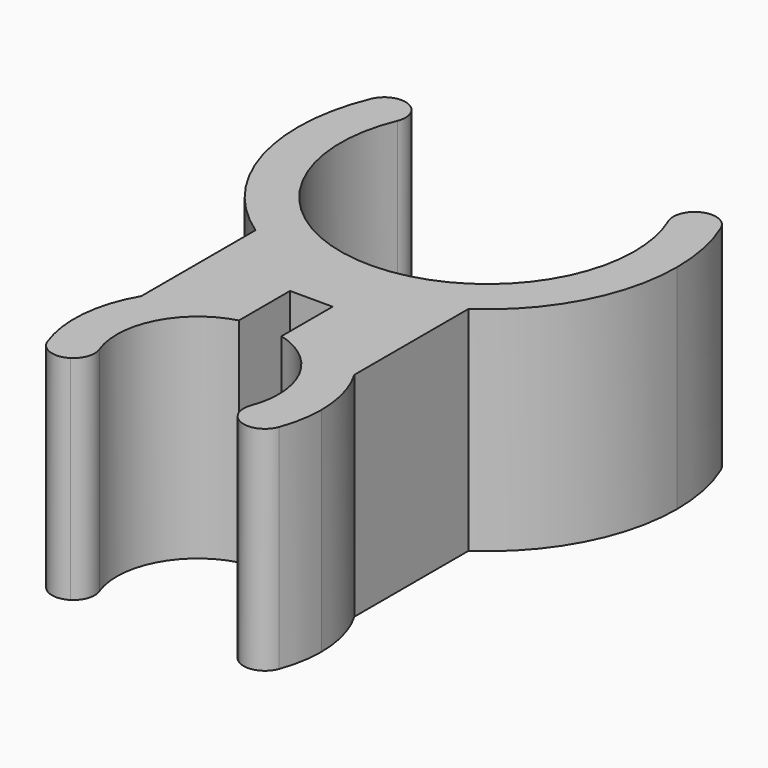
from build123d import *

# Parameters (mm, degrees)
F1_DEPTH = 10
F2_R     = 0.99999


# Not quite as in the source:
# - a fillet or chamfer is up to 0.001 mm smaller than in the source, because OpenCascade refuses the exact size


with BuildPart() as f1:
    # F0 (on Top) → F1 (new body)
    with BuildSketch(Plane.XY):
        with BuildLine():
            ThreePointArc((5.9755752861, 3.45), (6.6648882014, 1.7858514112), (6.9, 0))
            ThreePointArc((6.9, 0), (-1.7858514112, -6.6648882014), (-5.9755752861, 3.45))
            Line((-5.9755752861, 3.45), (-7.7076260937, 4.45))
            ThreePointArc((-7.7076260937, 4.45), (-8.6750314555, -1.9884238095), (-5, -7.3627440537))
            ThreePointArc((-5, -7.3627440537), (0, -8.9), (5, -7.3627440537))
            ThreePointArc((5, -7.3627440537), (7.8647949751, -4.1659332688), (8.9, 0))
            ThreePointArc((8.9, 0), (8.596739854, 2.3034895014), (7.7076260937, 4.45))
            Line((7.7076260937, 4.45), (5.9755752861, 3.45))
        make_face()
        with BuildLine():
            ThreePointArc((5, -7.3627440537), (0, -8.9), (-5, -7.3627440537))
            Line((-5, -7.3627440537), (-5, -14.0606123087))
            ThreePointArc((-5, -14.0606123087), (-3.30506116, -12.233809621), (-1, -11.2868572572))
            Line((-1, -11.2868572572), (-1, -10.333939444))
            Line((-1, -10.333939444), (1, -10.333939444))
            Line((1, -10.333939444), (1, -11.2868572572))
            ThreePointArc((1, -11.2868572572), (3.30506116, -12.233809621), (5, -14.0606123087))
            Line((5, -14.0606123087), (5, -7.3627440537))
        make_face()
        with BuildLine():
            ThreePointArc((-1, -11.2868572572), (-3.30506116, -12.233809621), (-5, -14.0606123087))
            ThreePointArc((-5, -14.0606123087), (-5.7990721969, -17.1037383981), (-4.8916703857, -20.1163377284))
            Line((-4.8916703857, -20.1163377284), (-3.2048874941, -19.0417385117))
            ThreePointArc((-3.2048874941, -19.0417385117), (-3.5447161041, -15.6306980825), (-1, -13.333939444))
            Line((-1, -13.333939444), (-1, -11.2868572572))
        make_face()
        with BuildLine():
            ThreePointArc((5.8, -17), (5.5964274319, -15.4768453788), (5, -14.0606123087))
            ThreePointArc((5, -14.0606123087), (3.30506116, -12.233809621), (1, -11.2868572572))
            Line((1, -11.2868572572), (1, -13.333939444))
            ThreePointArc((1, -13.333939444), (3.0199337741, -14.6934874811), (3.8, -17))
            ThreePointArc((3.8, -17), (3.6481894467, -18.0633502533), (3.2048874941, -19.0417385117))
            Line((3.2048874941, -19.0417385117), (4.8916703857, -20.1163377284))
            ThreePointArc((4.8916703857, -20.1163377284), (5.5682891554, -18.6230082814), (5.8, -17))
        make_face()
    extrude(amount=F1_DEPTH)

    # F2 (radius 1 in the source; OpenCascade refuses exactly that, so slightly less here)
    f2_edges = [f1.edges().sort_by_distance(p)[0] for p in [
        (-7.707626, 4.45, 5),
        (-5.975575, 3.45, 5),
        (5.975575, 3.45, 5),
        (7.707626, 4.45, 5),
        (-4.89167, -20.116338, 5),
        (-3.204887, -19.041739, 5),
        (4.89167, -20.116338, 5),
        (3.204887, -19.041739, 5),
    ]]
    fillet(f2_edges, radius=F2_R)


solid = f1.part
